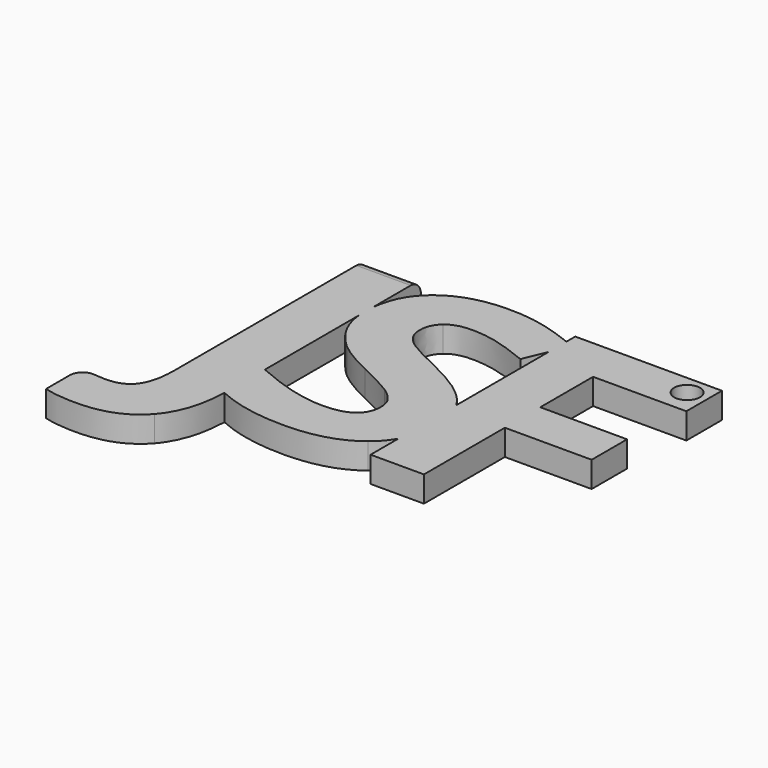
from build123d import *

# Parameters (mm, degrees)
F1_DEPTH = 2.54
F2_R     = 1.27
F3_DEPTH = 25.4
F4_R     = 1.27
F5_R     = 1.26999
F6_R     = 1.27


# Not quite as in the source:
# - a fillet or chamfer is up to 0.001 mm smaller than in the source, because OpenCascade refuses the exact size


with BuildPart() as f1:
    # F0 (on Top) → F1 (new body)
    with BuildSketch(Plane.XY):
        with BuildLine():
            add(Edge.make_bspline(
                [(-35.5870129937, -0.7740028705), (-37.3949991048, -0.7740028705), (-38.7399643826, -0.3936643288)],
                knots=[0, 0, 0, 1, 1, 1], degree=2))
            add(Edge.make_bspline(
                [(-29.6256197645, 1.5355891434), (-31.6403116048, -0.7740028705), (-35.5870129937, -0.7740028705)],
                knots=[0, 0, 0, 1, 1, 1], degree=2))
            add(Edge.make_bspline(
                [(-27.6205460855, 7.6555567964), (-27.750131484, 3.6856017003), (-29.6256197645, 1.5355891434)],
                knots=[0.0690942193, 0.0690942193, 0.0690942193, 1, 1, 1], degree=2))
            add(Edge.make_bspline(
                [(-27.6205460855, 7.6555567964), (-27.7827885359, 7.7299650226), (-27.9425390354, 7.8084190045)],
                knots=[0.9484314806, 0.9484314806, 0.9484314806, 1, 1, 1], degree=2))
            Line((-27.9425390354, 7.8084190045), (-27.9425390354, 12.7693565045))
            add(Edge.make_bspline(
                [(-27.9425390354, 12.7693565045), (-27.775046491, 12.6943111437), (-27.6109279243, 12.6221986399)],
                knots=[0, 0, 0, 0.0657706688, 0.0657706688, 0.0657706688], degree=2))
            Line((-27.6109279243, 12.6221986399), (-27.6109279243, 24.1901567001))
            add(Edge.make_bspline(
                [(-27.6109279243, 24.1901567001), (-27.6503949382, 24.5883728176), (-27.6503949382, 25.011847824)],
                knots=[0.7606675952, 0.7606675952, 0.7606675952, 1, 1, 1], degree=2))
            add(Edge.make_bspline(
                [(-27.6503949382, 25.011847824), (-27.6503949382, 25.4534645742), (-27.6109279243, 25.8700663435)],
                knots=[0, 0, 0, 0.1319883501, 0.1319883501, 0.1319883501], degree=2))
            Line((-27.6109279243, 25.8700663435), (-27.6109279243, 31.8193565045))
            Line((-27.6109279243, 31.8193565045), (-32.9522039659, 31.8193565045))
            Line((-32.9522039659, 31.8193565045), (-32.9522039659, 8.2218304629))
            add(Edge.make_bspline(
                [(-33.7101249729, 4.8015396643), (-32.9522039659, 5.8957019906), (-32.9522039659, 8.2218304629)],
                knots=[0, 0, 0, 1, 1, 1], degree=2))
            add(Edge.make_bspline(
                [(-36.2264227159, 3.7073773379), (-34.4680459798, 3.7073773379), (-33.7101249729, 4.8015396643)],
                knots=[0, 0, 0, 1, 1, 1], degree=2))
            add(Edge.make_bspline(
                [(-38.7399643826, 4.0491308101), (-37.3619261882, 3.7073773379), (-36.2264227159, 3.7073773379)],
                knots=[0, 0, 0, 1, 1, 1], degree=2))
            Line((-38.7399643826, 4.0491308101), (-38.7399643826, -0.3936643288))
        make_face()
        with BuildLine():
            add(Edge.make_bspline(
                [(-27.6205460855, 7.6555567964), (-27.7827885359, 7.7299650226), (-27.9425390354, 7.8084190045)],
                knots=[0.9484314806, 0.9484314806, 0.9484314806, 1, 1, 1], degree=2))
            add(Edge.make_bspline(
                [(-27.6109279243, 8.2549033795), (-27.6109279243, 7.9502170655), (-27.6205460855, 7.6555567964)],
                knots=[0, 0, 0, 0.0690942193, 0.0690942193, 0.0690942193], degree=2))
            Line((-27.6109279243, 8.2549033795), (-27.6109279243, 12.6221986399))
            add(Edge.make_bspline(
                [(-27.9425390354, 12.7693565045), (-27.775046491, 12.6943111437), (-27.6109279243, 12.6221986399)],
                knots=[0, 0, 0, 0.0657706688, 0.0657706688, 0.0657706688], degree=2))
            Line((-27.9425390354, 12.7693565045), (-27.9425390354, 7.8084190045))
        make_face()
        with BuildLine():
            add(Edge.make_bspline(
                [(-27.6109279243, 8.2549033795), (-27.6109279243, 7.9502170655), (-27.6205460855, 7.6555567964)],
                knots=[0, 0, 0, 0.0690942193, 0.0690942193, 0.0690942193], degree=2))
            add(Edge.make_bspline(
                [(-20.8098133409, 6.2870648379), (-24.63663557, 6.2870648379), (-27.6205460855, 7.6555567964)],
                knots=[0, 0, 0, 0.9484314806, 0.9484314806, 0.9484314806], degree=2))
            add(Edge.make_bspline(
                [(-13.9830121257, 8.2521473031), (-16.4386761882, 6.2870648379), (-20.8098133409, 6.2870648379)],
                knots=[0, 0, 0, 1, 1, 1], degree=2))
            add(Edge.make_bspline(
                [(-12.4203168132, 10.0403583252), (-13.0081692098, 9.0322404558), (-13.9830121257, 8.2521473031)],
                knots=[0.6030226892, 0.6030226892, 0.6030226892, 1, 1, 1], degree=2))
            Line((-12.4203168132, 10.0403583252), (-12.4203168132, 17.1746575044))
            add(Edge.make_bspline(
                [(-12.8364843479, 17.7881716087), (-12.6085593245, 17.4930686838), (-12.4203168132, 17.1746575044)],
                knots=[0, 0, 0, 0.1741033581, 0.1741033581, 0.1741033581], degree=2))
            add(Edge.make_bspline(
                [(-17.6789105632, 21.1753894906), (-14.1456206326, 19.4831585879), (-12.8364843479, 17.7881716087)],
                knots=[0, 0, 0, 1, 1, 1], degree=2))
            add(Edge.make_bspline(
                [(-21.0606162923, 22.9392783795), (-20.3467925076, 22.4486967823), (-17.6789105632, 21.1753894906)],
                knots=[0, 0, 0, 1, 1, 1], degree=2))
            add(Edge.make_bspline(
                [(-22.1024131673, 23.956270567), (-21.774440077, 23.4298599768), (-21.0606162923, 22.9392783795)],
                knots=[0, 0, 0, 1, 1, 1], degree=2))
            add(Edge.make_bspline(
                [(-22.4303862576, 25.1882367129), (-22.4303862576, 24.4826811573), (-22.1024131673, 23.956270567)],
                knots=[0, 0, 0, 1, 1, 1], degree=2))
            add(Edge.make_bspline(
                [(-21.6200997993, 27.0292957406), (-22.4303862576, 26.3237401851), (-22.4303862576, 25.1882367129)],
                knots=[0, 0, 0, 1, 1, 1], degree=2))
            add(Edge.make_bspline(
                [(-19.293971327, 27.7348512962), (-20.8098133409, 27.7348512962), (-21.6200997993, 27.0292957406)],
                knots=[0, 0, 0, 1, 1, 1], degree=2))
            add(Edge.make_bspline(
                [(-16.7032595215, 27.4068782059), (-18.0206640354, 27.7348512962), (-19.293971327, 27.7348512962)],
                knots=[0, 0, 0, 1, 1, 1], degree=2))
            add(Edge.make_bspline(
                [(-13.3684070909, 26.252082199), (-15.3858550076, 27.0789051156), (-16.7032595215, 27.4068782059)],
                knots=[0, 0, 0, 1, 1, 1], degree=2))
            Line((-13.3684070909, 26.252082199), (-12.4203168132, 28.5433003703))
            Line((-12.4203168132, 28.5433003703), (-12.4203168132, 30.7303313899))
            add(Edge.make_bspline(
                [(-15.3775867784, 31.7146256018), (-13.9509902659, 31.3441955954), (-12.4203168132, 30.7303313899)],
                knots=[0, 0, 0, 0.8000288101, 0.8000288101, 0.8000288101], degree=2))
            add(Edge.make_bspline(
                [(-19.1230945909, 32.1776464351), (-17.160768202, 32.1776464351), (-15.3775867784, 31.7146256018)],
                knots=[0, 0, 0, 1, 1, 1], degree=2))
            add(Edge.make_bspline(
                [(-25.3849001465, 30.2676854976), (-23.1194053548, 32.1776464351), (-19.1230945909, 32.1776464351)],
                knots=[0, 0, 0, 1, 1, 1], degree=2))
            add(Edge.make_bspline(
                [(-27.6109279243, 25.8700663435), (-27.3513760183, 28.6098171531), (-25.3849001465, 30.2676854976)],
                knots=[0.1319883501, 0.1319883501, 0.1319883501, 1, 1, 1], degree=2))
            Line((-27.6109279243, 25.8700663435), (-27.6109279243, 24.1901567001))
            add(Edge.make_bspline(
                [(-26.9613758409, 21.9140179629), (-27.4854903406, 22.9245107183), (-27.6109279243, 24.1901567001)],
                knots=[0, 0, 0, 0.7606675952, 0.7606675952, 0.7606675952], degree=2))
            add(Edge.make_bspline(
                [(-25.1175607368, 19.5878894906), (-26.2723567437, 20.5855891434), (-26.9613758409, 21.9140179629)],
                knots=[0, 0, 0, 1, 1, 1], degree=2))
            add(Edge.make_bspline(
                [(-21.6586848687, 17.5042957406), (-23.9627647298, 18.5901898379), (-25.1175607368, 19.5878894906)],
                knots=[0, 0, 0, 1, 1, 1], degree=2))
            add(Edge.make_bspline(
                [(-18.3927343479, 15.7982844559), (-19.194752577, 16.330207199), (-21.6586848687, 17.5042957406)],
                knots=[0, 0, 0, 1, 1, 1], degree=2))
            add(Edge.make_bspline(
                [(-17.1773046604, 14.6875856712), (-17.5907161187, 15.2663617129), (-18.3927343479, 15.7982844559)],
                knots=[0, 0, 0, 1, 1, 1], degree=2))
            add(Edge.make_bspline(
                [(-16.763893202, 13.3701811573), (-16.763893202, 14.1088096295), (-17.1773046604, 14.6875856712)],
                knots=[0, 0, 0, 1, 1, 1], degree=2))
            add(Edge.make_bspline(
                [(-17.7037152507, 11.3720257754), (-16.763893202, 12.0417523379), (-16.763893202, 13.3701811573)],
                knots=[0, 0, 0, 1, 1, 1], degree=2))
            add(Edge.make_bspline(
                [(-20.3964018826, 10.7022992129), (-18.6435372993, 10.7022992129), (-17.7037152507, 11.3720257754)],
                knots=[0, 0, 0, 1, 1, 1], degree=2))
            add(Edge.make_bspline(
                [(-23.6292794868, 11.1653200462), (-21.8626345215, 10.7022992129), (-20.3964018826, 10.7022992129)],
                knots=[0, 0, 0, 1, 1, 1], degree=2))
            add(Edge.make_bspline(
                [(-27.6109279243, 12.6221986399), (-25.2797310311, 11.5978876896), (-23.6292794868, 11.1653200462)],
                knots=[0.0657706688, 0.0657706688, 0.0657706688, 1, 1, 1], degree=2))
            Line((-27.6109279243, 12.6221986399), (-27.6109279243, 8.2549033795))
        make_face()
        with BuildLine():
            add(Edge.make_bspline(
                [(-27.6109279243, 24.1901567001), (-27.6503949382, 24.5883728176), (-27.6503949382, 25.011847824)],
                knots=[0.7606675952, 0.7606675952, 0.7606675952, 1, 1, 1], degree=2))
            Line((-27.6109279243, 24.1901567001), (-27.6109279243, 25.8700663435))
            add(Edge.make_bspline(
                [(-27.6503949382, 25.011847824), (-27.6503949382, 25.4534645742), (-27.6109279243, 25.8700663435)],
                knots=[0, 0, 0, 0.1319883501, 0.1319883501, 0.1319883501], degree=2))
        make_face()
        with BuildLine():
            Line((-12.4203168132, 17.1746575044), (-12.4203168132, 10.0403583252))
            add(Edge.make_bspline(
                [(-11.5273480632, 13.6292523379), (-11.5273480632, 11.5717253126), (-12.4203168132, 10.0403583252)],
                knots=[0, 0, 0, 0.6030226892, 0.6030226892, 0.6030226892], degree=2))
            add(Edge.make_bspline(
                [(-12.4203168132, 17.1746575044), (-11.5273480632, 15.6642057435), (-11.5273480632, 13.6292523379)],
                knots=[0.1741033581, 0.1741033581, 0.1741033581, 1, 1, 1], degree=2))
        make_face()
        with BuildLine():
            add(Edge.make_bspline(
                [(-11.5273480632, 13.6292523379), (-11.5273480632, 11.5717253126), (-12.4203168132, 10.0403583252)],
                knots=[0, 0, 0, 0.6030226892, 0.6030226892, 0.6030226892], degree=2))
            Line((-12.4203168132, 10.0403583252), (-12.4203168132, 6.6343304629))
            Line((-12.4203168132, 6.6343304629), (-7.1672352159, 6.6343304629))
            Line((-7.1672352159, 6.6343304629), (-7.1672352159, 16.5892783795))
            Line((-7.1672352159, 16.5892783795), (1.3766015896, 16.5892783795))
            Line((1.3766015896, 16.5892783795), (1.3766015896, 20.9493912268))
            Line((1.3766015896, 20.9493912268), (-7.1672352159, 20.9493912268))
            Line((-7.1672352159, 20.9493912268), (-7.1672352159, 27.442707199))
            Line((-7.1672352159, 27.442707199), (2.0160113118, 27.442707199))
            Line((2.0160113118, 27.442707199), (2.0160113118, 31.8193565045))
            Line((2.0160113118, 31.8193565045), (-12.4203168132, 31.8193565045))
            Line((-12.4203168132, 31.8193565045), (-12.4203168132, 30.7303313899))
            add(Edge.make_bspline(
                [(-12.4203168132, 30.7303313899), (-12.037717352, 30.5768929712), (-11.6486154243, 30.4082453934)],
                knots=[0.8000288101, 0.8000288101, 0.8000288101, 1, 1, 1], degree=2))
            Line((-11.6486154243, 30.4082453934), (-12.4203168132, 28.5433003703))
            Line((-12.4203168132, 28.5433003703), (-12.4203168132, 17.1746575044))
            add(Edge.make_bspline(
                [(-12.4203168132, 17.1746575044), (-11.5273480632, 15.6642057435), (-11.5273480632, 13.6292523379)],
                knots=[0.1741033581, 0.1741033581, 0.1741033581, 1, 1, 1], degree=2))
        make_face()
        with BuildLine():
            Line((-12.4203168132, 30.7303313899), (-12.4203168132, 28.5433003703))
            Line((-12.4203168132, 28.5433003703), (-11.6486154243, 30.4082453934))
            add(Edge.make_bspline(
                [(-12.4203168132, 30.7303313899), (-12.037717352, 30.5768929712), (-11.6486154243, 30.4082453934)],
                knots=[0.8000288101, 0.8000288101, 0.8000288101, 1, 1, 1], degree=2))
        make_face()
    extrude(amount=F1_DEPTH)

    # F2 (on face) → F3 (cut)
    with BuildSketch(Plane.XY.offset(2.54)):
        with Locations((0.1110113118, 29.9143565045)):
            Circle(F2_R)
    extrude(amount=-F3_DEPTH, mode=Mode.SUBTRACT)

    # F4
    f4_edges = [f1.edges().sort_by_distance(p)[0] for p in [
        (-30.281566, 31.819357, 2.54),
    ]]
    fillet(f4_edges, radius=F4_R)

    # F5 (radius 1.27 in the source; OpenCascade refuses exactly that, so slightly less here)
    f5_edges = [f1.edges().sort_by_distance(p)[0] for p in [
        (-30.281566, 31.819357, 0),
    ]]
    fillet(f5_edges, radius=F5_R)

    # F6
    f6_edges = [f1.edges().sort_by_distance(p)[0] for p in [
        (-38.739964, 4.049131, 1.27),
    ]]
    fillet(f6_edges, radius=F6_R)


solid = f1.part
